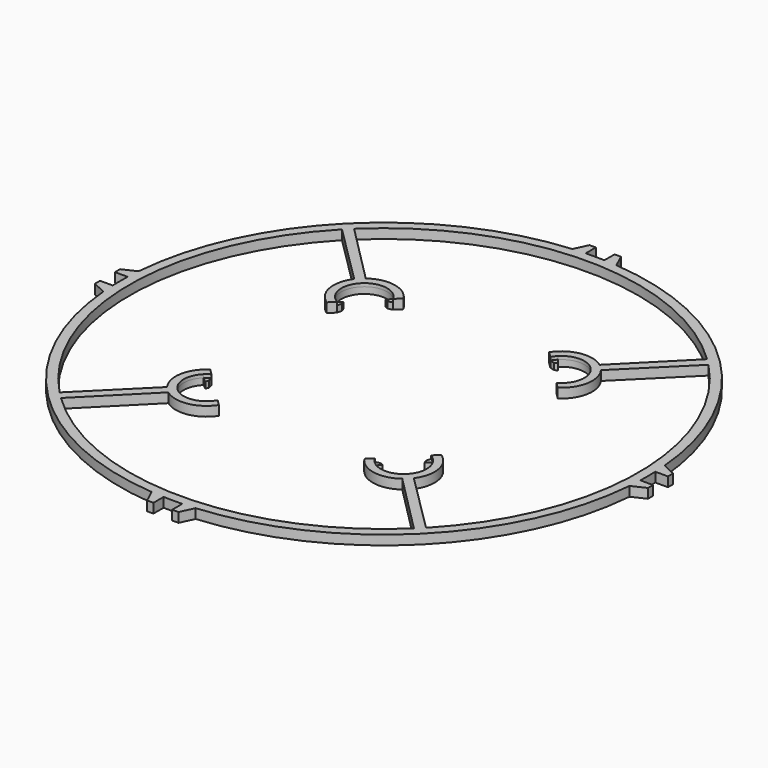
from build123d import *
from build123d import SkipClean  # not in build123d's __all__

# Parameters (mm, degrees)
F1_R     = 41.5
F3_DEPTH = 1.5
F4_DEPTH = 1.5
F5_R     = 3.6
F6_DEPTH = 0.5


with BuildPart() as f3:
    # F1 (on face) → F3 (new body)
    with BuildSketch(Plane.XY):
        Circle(F1_R)
        with BuildLine():
            Line((-17.2474476501, 12.3525523499), (-17.0531188132, 13.0769391962))
            Line((-17.0531188132, 13.0769391962), (-17.2364935, 13.5420990873))
            Line((-17.2364935, 13.5420990873), (-18.0455844123, 12.9544155877))
            ThreePointArc((-18.0455844123, 12.9544155877), (-18.0455844123, 18.0455844123), (-12.9544155877, 18.0455844123))
            Line((-12.9544155877, 18.0455844123), (-13.5420990873, 17.2364935))
            Line((-13.5420990873, 17.2364935), (-13.0769391962, 17.0531188132))
            Line((-13.0769391962, 17.0531188132), (-12.3525523499, 17.2474476501))
            Line((-12.3525523499, 17.2474476501), (-11.442760334, 18.1573118546))
            ThreePointArc((-11.442760334, 18.1573118546), (-14.6482964144, 20.2746309807), (-18.3882088979, 19.3962481135))
            Line((-18.3882088979, 19.3962481135), (-27.7493051541, 28.8093051541))
            ThreePointArc((-27.7493051541, 28.8093051541), (0, 40), (27.7493051541, 28.8093051541))
            Line((27.7493051541, 28.8093051541), (18.3882088979, 19.3962481135))
            ThreePointArc((18.3882088979, 19.3962481135), (14.6483525281, 20.27464099), (11.442822795, 18.1574072189))
            Line((11.442822795, 18.1574072189), (12.3525523499, 17.2474476501))
            Line((12.3525523499, 17.2474476501), (13.0769391962, 17.0531188132))
            Line((13.0769391962, 17.0531188132), (13.5420990873, 17.2364935))
            Line((13.5420990873, 17.2364935), (12.9544155877, 18.0455844123))
            ThreePointArc((12.9544155877, 18.0455844123), (18.0455844123, 18.0455844123), (18.0455844123, 12.9544155877))
            Line((18.0455844123, 12.9544155877), (17.2364935, 13.5420990873))
            Line((17.2364935, 13.5420990873), (17.0531188132, 13.0769391962))
            Line((17.0531188132, 13.0769391962), (17.2474476501, 12.3525523499))
            Line((17.2474476501, 12.3525523499), (18.1573118546, 11.442760334))
            ThreePointArc((18.1573118546, 11.442760334), (20.2746309807, 14.6482964144), (19.3962481135, 18.3882088979))
            Line((19.3962481135, 18.3882088979), (28.8093051541, 27.7493051541))
            ThreePointArc((28.8093051541, 27.7493051541), (40, 0), (28.8093051541, -27.7493051541))
            Line((28.8093051541, -27.7493051541), (19.3962481135, -18.3882088979))
            ThreePointArc((19.3962481135, -18.3882088979), (20.27464099, -14.6483525281), (18.1574072189, -11.442822795))
            Line((18.1574072189, -11.442822795), (17.2474476501, -12.3525523499))
            Line((17.2474476501, -12.3525523499), (17.0531188132, -13.0769391962))
            Line((17.0531188132, -13.0769391962), (17.2364935, -13.5420990873))
            Line((17.2364935, -13.5420990873), (18.0455844123, -12.9544155877))
            ThreePointArc((18.0455844123, -12.9544155877), (18.0455844123, -18.0455844123), (12.9544155877, -18.0455844123))
            Line((12.9544155877, -18.0455844123), (13.5420990873, -17.2364935))
            Line((13.5420990873, -17.2364935), (13.0769391962, -17.0531188132))
            Line((13.0769391962, -17.0531188132), (12.3525523499, -17.2474476501))
            Line((12.3525523499, -17.2474476501), (11.442760334, -18.1573118546))
            ThreePointArc((11.442760334, -18.1573118546), (14.6482964144, -20.2746309807), (18.3882088979, -19.3962481135))
            Line((18.3882088979, -19.3962481135), (27.7493051541, -28.8093051541))
            ThreePointArc((27.7493051541, -28.8093051541), (0, -40), (-27.7493051541, -28.8093051541))
            Line((-27.7493051541, -28.8093051541), (-18.3882088979, -19.3962481135))
            ThreePointArc((-18.3882088979, -19.3962481135), (-14.6483525281, -20.27464099), (-11.442822795, -18.1574072189))
            Line((-11.442822795, -18.1574072189), (-12.3525523499, -17.2474476501))
            Line((-12.3525523499, -17.2474476501), (-13.0769391962, -17.0531188132))
            Line((-13.0769391962, -17.0531188132), (-13.5420990873, -17.2364935))
            Line((-13.5420990873, -17.2364935), (-12.9544155877, -18.0455844123))
            ThreePointArc((-12.9544155877, -18.0455844123), (-18.0455844123, -18.0455844123), (-18.0455844123, -12.9544155877))
            Line((-18.0455844123, -12.9544155877), (-17.2364935, -13.5420990873))
            Line((-17.2364935, -13.5420990873), (-17.0531188132, -13.0769391962))
            Line((-17.0531188132, -13.0769391962), (-17.2474476501, -12.3525523499))
            Line((-17.2474476501, -12.3525523499), (-18.1573118546, -11.442760334))
            ThreePointArc((-18.1573118546, -11.442760334), (-20.2746309807, -14.6482964144), (-19.3962481135, -18.3882088979))
            Line((-19.3962481135, -18.3882088979), (-28.8093051541, -27.7493051541))
            ThreePointArc((-28.8093051541, -27.7493051541), (-40, 0), (-28.8093051541, 27.7493051541))
            Line((-28.8093051541, 27.7493051541), (-19.3962481135, 18.3882088979))
            ThreePointArc((-19.3962481135, 18.3882088979), (-20.27464099, 14.6483525281), (-18.1574072189, 11.442822795))
            Line((-18.1574072189, 11.442822795), (-17.2474476501, 12.3525523499))
        make_face(mode=Mode.SUBTRACT)
    extrude(amount=F3_DEPTH)

    # F2 (on Top) → F4 (join)
    with BuildSketch(Plane.XY):
        Polygon((-1.47, 41.4739568886), (-1.47, 43.4739568886), (-2.47, 43.4739568886), (-3.4575279787, 41.3557190758), align=None)
        Polygon((2.47, 43.4739568886), (1.47, 43.4739568886), (1.47, 41.4739568886), (3.4575279787, 41.3557190758), align=None)
        Polygon((-43.4739568886, 2.47), (-43.4739568886, 1.47), (-41.4739568886, 1.47), (-41.3557190758, 3.4575279787), align=None)
        Polygon((-41.4739568886, -1.47), (-43.4739568886, -1.47), (-43.4739568886, -2.47), (-41.3557190758, -3.4575279787), align=None)
        Polygon((-2.47, -43.4739568886), (-1.47, -43.4739568886), (-1.47, -41.4739568886), (-3.4575279787, -41.3557190758), align=None)
        Polygon((1.47, -41.4739568886), (1.47, -43.4739568886), (2.47, -43.4739568886), (3.4575279787, -41.3557190758), align=None)
        Polygon((43.4739568886, -2.47), (43.4739568886, -1.47), (41.4739568886, -1.47), (41.3557190758, -3.4575279787), align=None)
        Polygon((41.4739568886, 1.47), (43.4739568886, 1.47), (43.4739568886, 2.47), (41.3557190758, 3.4575279787), align=None)
    extrude(amount=F4_DEPTH)

    # F5 (on face) → F6 (cut)
    with BuildSketch(Plane.XY.offset(1.5)):
        with Locations((-15.5, 15.5)):
            Circle(F5_R)
        with Locations((-15.5, -15.5)):
            Circle(F5_R)
        with Locations((15.5, -15.5)):
            Circle(F5_R)
        with Locations((15.5, 15.5)):
            Circle(F5_R)
    with SkipClean():  # cleaning this boolean's faces spoils the solid; the shape is the same uncleaned
        extrude(amount=-F6_DEPTH, mode=Mode.SUBTRACT)


solid = f3.part
